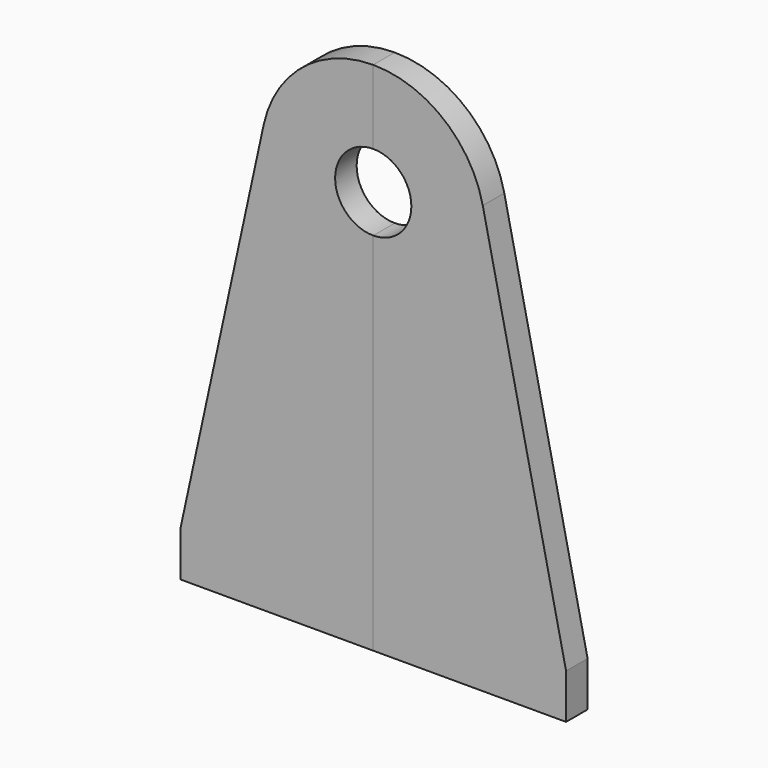
from build123d import *
from build123d import SkipClean  # not in build123d's __all__

# Parameters (mm, degrees)
F1_DEPTH = 6


with BuildPart() as f1:
    # F0 (on Front) → F1 (new body)
    with BuildSketch(Plane.XZ):
        with BuildLine():
            Line((-43, 0), (0, 0))
            Line((0, 0), (0, 81.5))
            ThreePointArc((0, 81.5), (-8.5, 90), (0, 98.5))
            Line((0, 98.5), (0, 115))
            ThreePointArc((0, 115), (-15.6853772226, 109.4671246306), (-24.4279354617, 95.3175153107))
            Line((-24.4279354617, 95.3175153107), (-43, 10))
            Line((-43, 10), (-43, 0))
        make_face()
    extrude(amount=F1_DEPTH)

    # F2: F1 across plane


with BuildPart() as f1_1:
    add(f1.part, clean=False)
    with SkipClean():  # cleaning this boolean's faces spoils the solid; the shape is the same uncleaned
        add(f1.part.mirror(Plane.YZ), clean=False)


solid = f1_1.part
